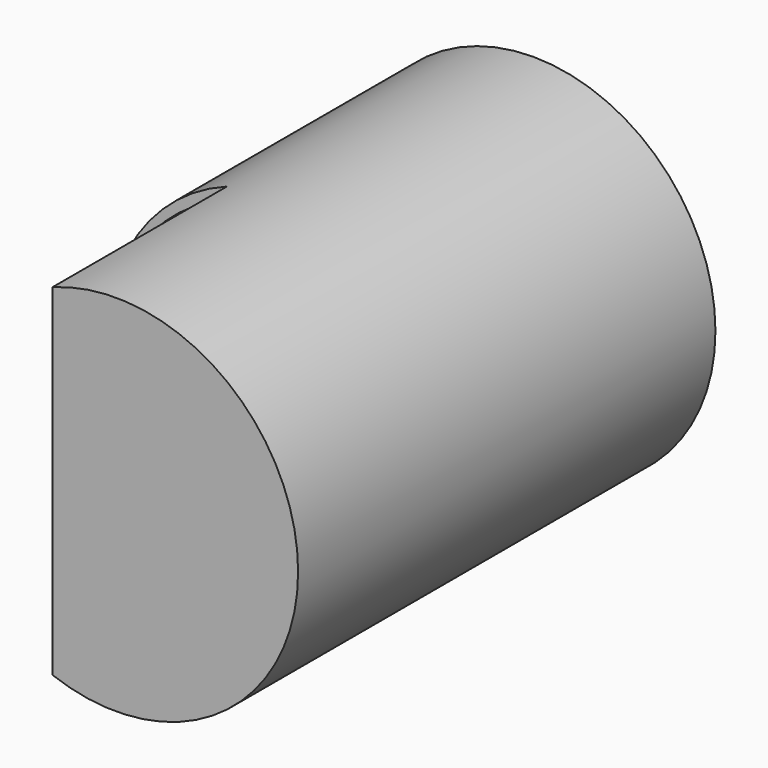
from build123d import *

# Parameters (mm, degrees)
F0_R     = 31.0947263036
F1_DEPTH = 89.0598669648
F3_DEPTH = 37.2095629573
F5_DEPTH = 51.1443465948


with BuildPart() as f1:
    # F0 (on Front) → F1 (new body)
    with BuildSketch(Plane.XZ):
        Circle(F0_R)
    extrude(amount=F1_DEPTH)

    # F2 (on face) → F3 (cut)
    with BuildSketch(Plane.XZ.offset(89.0598669648)):
        with BuildLine():
            Line((-10.8266547322, -29.1490231604), (-10.8266547322, 0))
            Line((-10.8266547322, 0), (-10.8266547322, 29.1490231604))
            ThreePointArc((-10.8266547322, 29.1490231604), (-31.0947263036, 0), (-10.8266547322, -29.1490231604))
        make_face()
    extrude(amount=-F3_DEPTH, mode=Mode.SUBTRACT)

    # F4 (on face) → F5 (cut)
    with BuildSketch(Plane.XZ.offset(51.8503040075)):
        with BuildLine():
            Line((-10.8266547322, -28.2442569733), (-10.8266547322, 27.0338580012))
            ThreePointArc((-10.8266547322, 27.0338580012), (-30.3341260618, -0.605199486), (-10.8266547322, -28.2442569733))
        make_face()
    extrude(amount=-F5_DEPTH, mode=Mode.SUBTRACT)


solid = f1.part
